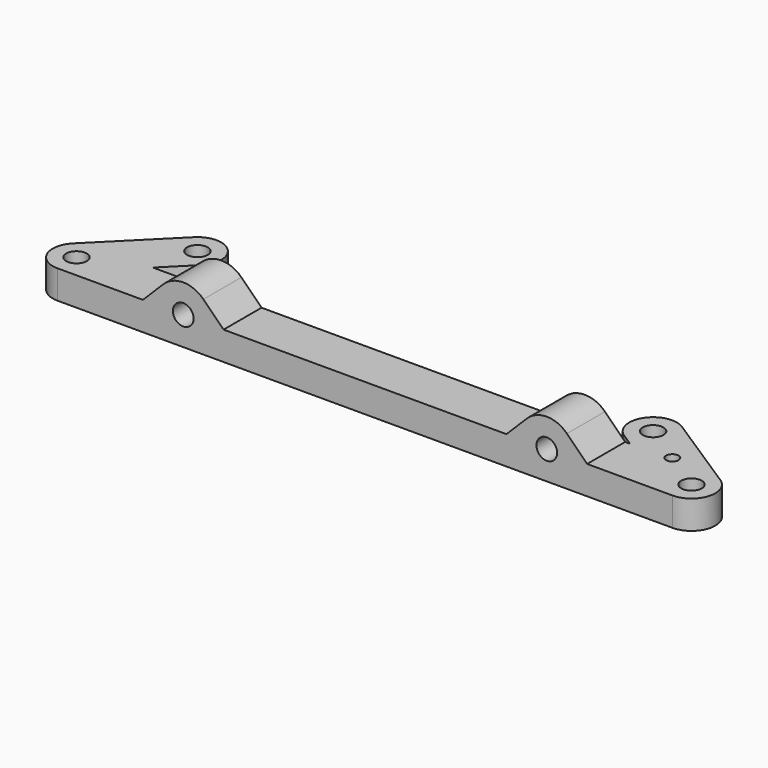
from build123d import *

# Parameters (mm, degrees)
F0_R     = 1.7272
F0_R_2   = 1.0407250193
F1_DEPTH = 4.7625
F3_DEPTH = 7.9375
F4_R     = 1.7272
F5_DEPTH = 7.9375


with BuildPart() as f1:
    # F0 (on Top) → F1 (new body)
    with BuildSketch(Plane.XY):
        with BuildLine():
            Line((-2.0541653616, 1.330521752), (0, 0))
            Line((0, 0), (-79.738154648, 0))
            Line((-79.738154648, 0), (-75.2879145345, 4.4502401135))
            ThreePointArc((-75.2879145345, 4.4502401135), (-75.2879145345, 10.0629001892), (-80.9005746101, 10.0629001892))
            Line((-80.9005746101, 10.0629001892), (-92.1258947615, -1.1624199622))
            ThreePointArc((-92.1258947615, -1.1624199622), (-92.9862116183, -5.4875248722), (-89.3195647236, -7.9375))
            Line((-89.3195647236, -7.9375), (13.4275761574, -7.9375))
            ThreePointArc((13.4275761574, -7.9375), (17.2335612406, -5.093674046), (15.5851543061, -0.6377091574))
            Line((15.5851543061, -0.6377091574), (2.2609909357, 7.9926034372))
            ThreePointArc((2.2609909357, 7.9926034372), (-3.2276280555, 6.8191407432), (-2.0541653616, 1.330521752))
        make_face()
        with Locations((-89.3195647236, -3.96875)):
            Circle(F0_R, mode=Mode.SUBTRACT)
        with Locations((13.4275761574, -3.96875)):
            Circle(F0_R, mode=Mode.SUBTRACT)
        with Locations((6.7654944722, 0.3464062973)):
            Circle(F0_R_2, mode=Mode.SUBTRACT)
        with Locations((-78.0942445723, 7.2565701513)):
            Circle(F0_R, mode=Mode.SUBTRACT)
        with Locations((0.1034127871, 4.6615625946)):
            Circle(F0_R, mode=Mode.SUBTRACT)
    extrude(amount=F1_DEPTH)

    # F2 (on face) → F3 (join, through all)
    with BuildSketch(Plane.XZ.offset(7.9375)):
        with BuildLine():
            Line((-75.0487659739, 4.7625), (-68.3135738831, 4.7625))
            Line((-68.3135738831, 4.7625), (-61.5783817923, 4.7625))
            Line((-61.5783817923, 4.7625), (-64.9459778377, 8.1300960454))
            ThreePointArc((-64.9459778377, 8.1300960454), (-68.3135738831, 9.525), (-71.6811699285, 8.1300960454))
            Line((-71.6811699285, 8.1300960454), (-75.0487659739, 4.7625))
        make_face()
        with BuildLine():
            Line((-14.3136067739, 4.7625), (-7.5784146831, 4.7625))
            Line((-7.5784146831, 4.7625), (-0.8432225923, 4.7625))
            Line((-0.8432225923, 4.7625), (-4.2108186377, 8.1300960454))
            ThreePointArc((-4.2108186377, 8.1300960454), (-7.5784146831, 9.525), (-10.9460107285, 8.1300960454))
            Line((-10.9460107285, 8.1300960454), (-14.3136067739, 4.7625))
        make_face()
    extrude(amount=-F3_DEPTH)

    # F4 (on face) → F5 (cut, through all)
    with BuildSketch(Plane.XZ.offset(7.9375)):
        with Locations((-68.3135738831, 4.7625)):
            Circle(F4_R)
        with Locations((-7.5784146831, 4.7625)):
            Circle(F4_R)
    extrude(amount=-F5_DEPTH, mode=Mode.SUBTRACT)


solid = f1.part
